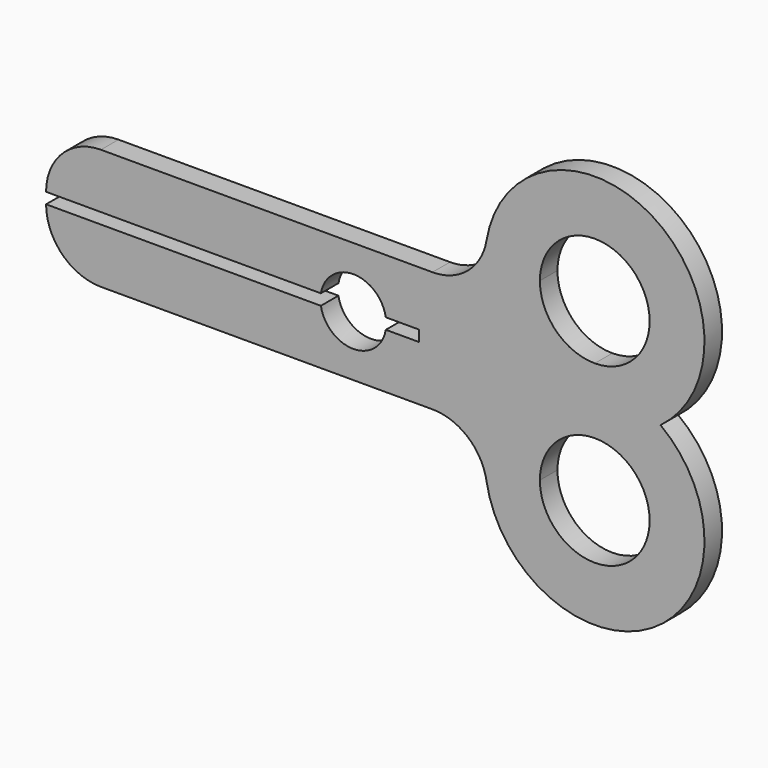
from build123d import *

# Parameters (mm, degrees)
F1_DEPTH = 2
F2_R     = 5
F4_DEPTH = 2


# Not quite as in the source:
# - a feature names something its author has since deleted; it is built from what else it names


with BuildPart() as f1:
    # F0 (on Front) → F1 (new body)
    with BuildSketch(Plane.XZ):
        with BuildLine():
            Line((0, 5.5), (0, 0))
            Line((0, 0), (40, 0))
            Line((40, 0), (40, 5.5))
            Line((40, 5.5), (31, 5.5))
            ThreePointArc((31, 5.5), (28, 2.5), (25, 5.5))
            Line((25, 5.5), (0, 5.5))
        make_face()
        with BuildLine():
            Line((40, 5.5), (40, 0))
            Line((40, 0), (40, -2.5))
            ThreePointArc((40, -2.5), (41.05572809, 1.972135955), (44, 5.5))
            Line((44, 5.5), (40, 5.5))
        make_face()
        with BuildLine():
            Line((0, 11), (0, 5.5))
            Line((0, 5.5), (25, 5.5))
            ThreePointArc((25, 5.5), (28, 8.5), (31, 5.5))
            Line((31, 5.5), (40, 5.5))
            Line((40, 5.5), (40, 11))
            Line((40, 11), (0, 11))
        make_face()
        with BuildLine():
            Line((40, 11), (40, 5.5))
            Line((40, 5.5), (44, 5.5))
            ThreePointArc((44, 5.5), (41.05572809, 9.027864045), (40, 13.5))
            Line((40, 13.5), (40, 11))
        make_face()
        with BuildLine():
            Line((45, -2.5), (40, -2.5))
            ThreePointArc((40, -2.5), (50, -12.5), (60, -2.5))
            ThreePointArc((60, -2.5), (58.94427191, 1.972135955), (56, 5.5))
            ThreePointArc((56, 5.5), (53.1622776602, 4.0131670195), (50, 3.5))
            Line((50, 3.5), (50, 2.5))
            ThreePointArc((50, 2.5), (53.5355339059, 1.0355339059), (55, -2.5))
            ThreePointArc((55, -2.5), (50, -7.5), (45, -2.5))
        make_face()
        with BuildLine():
            ThreePointArc((44, 5.5), (41.05572809, 1.972135955), (40, -2.5))
            Line((40, -2.5), (45, -2.5))
            ThreePointArc((45, -2.5), (46.4644660941, 1.0355339059), (50, 2.5))
            Line((50, 2.5), (50, 3.5))
            ThreePointArc((50, 3.5), (46.8377223398, 4.0131670195), (44, 5.5))
        make_face()
        with BuildLine():
            ThreePointArc((40, 13.5), (41.05572809, 9.027864045), (44, 5.5))
            ThreePointArc((44, 5.5), (46.8377223398, 6.9868329805), (50, 7.5))
            Line((50, 7.5), (50, 8.5))
            ThreePointArc((50, 8.5), (46.4644660941, 9.9644660941), (45, 13.5))
            Line((45, 13.5), (40, 13.5))
        make_face()
        with BuildLine():
            Line((50, 5.5), (44, 5.5))
            ThreePointArc((44, 5.5), (46.8377223398, 4.0131670195), (50, 3.5))
            Line((50, 3.5), (50, 5.5))
        make_face()
        with BuildLine():
            ThreePointArc((50, 7.5), (46.8377223398, 6.9868329805), (44, 5.5))
            Line((44, 5.5), (50, 5.5))
            Line((50, 5.5), (50, 7.5))
        make_face()
        with BuildLine():
            ThreePointArc((60, 13.5), (50, 23.5), (40, 13.5))
            Line((40, 13.5), (45, 13.5))
            ThreePointArc((45, 13.5), (50, 18.5), (55, 13.5))
            ThreePointArc((55, 13.5), (53.5355339059, 9.9644660941), (50, 8.5))
            Line((50, 8.5), (50, 7.5))
            ThreePointArc((50, 7.5), (53.1622776602, 6.9868329805), (56, 5.5))
            ThreePointArc((56, 5.5), (58.94427191, 9.027864045), (60, 13.5))
        make_face()
        with BuildLine():
            ThreePointArc((56, 5.5), (53.1622776602, 6.9868329805), (50, 7.5))
            Line((50, 7.5), (50, 5.5))
            Line((50, 5.5), (56, 5.5))
        make_face()
        with BuildLine():
            Line((50, 5.5), (50, 3.5))
            ThreePointArc((50, 3.5), (53.1622776602, 4.0131670195), (56, 5.5))
            Line((56, 5.5), (50, 5.5))
        make_face()
    extrude(amount=F1_DEPTH)

    # F2
    f2_edges = [f1.edges().sort_by_distance(p)[0] for p in [
        (40, -1, 11),
        (40, -1, 0),
        (0, -1, 11),
        (0, -1, 0),
    ]]
    fillet(f2_edges, radius=F2_R)

    # F3 (on face) → F4 (cut, through all)
    with BuildSketch(Plane.XZ.offset(2)):
        with BuildLine():
            Line((25.0419601085, 6), (0, 6))
            Line((0, 6), (0, 5))
            Line((0, 5), (25.0419601085, 5))
            ThreePointArc((25.0419601085, 5), (25, 5.5), (25.0419601085, 6))
        make_face()
        with BuildLine():
            Line((34, 6), (30.9580398915, 6))
            ThreePointArc((30.9580398915, 6), (30.9894915684, 5.7508787808), (31, 5.5))
            ThreePointArc((31, 5.5), (30.9894915684, 5.2491212192), (30.9580398915, 5))
            Line((30.9580398915, 5), (34, 5))
            Line((34, 5), (34, 6))
        make_face()
    extrude(amount=-F4_DEPTH, mode=Mode.SUBTRACT)


solid = f1.part
